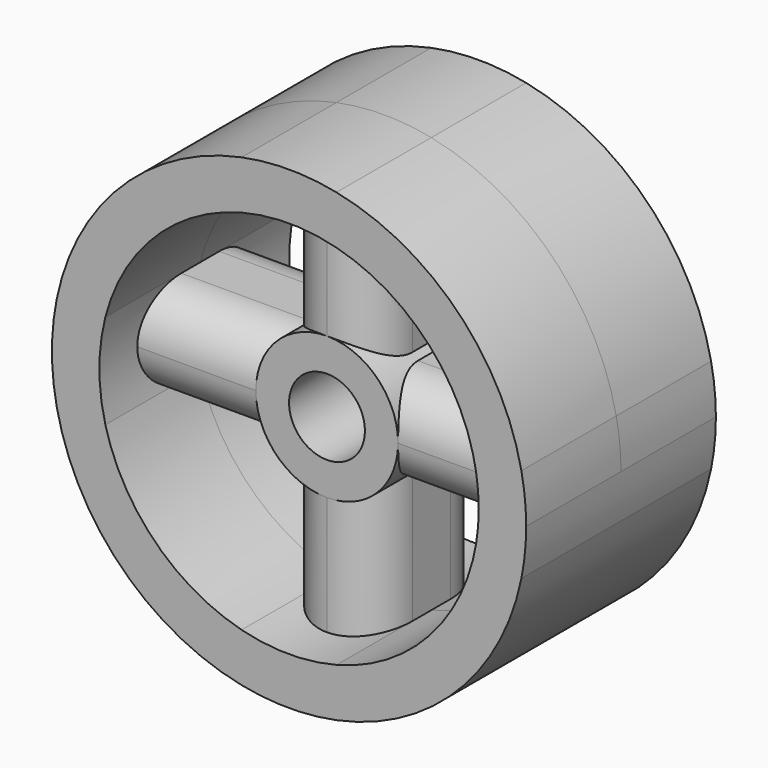
from build123d import *

# Parameters (mm, degrees)
F1_DEPTH = 12.5
F0_R     = 4
F2_DEPTH = 7.5
F3_R     = 4.99999
F4_R     = 4.99999


# Not quite as in the source:
# - a fillet or chamfer is up to 0.001 mm smaller than in the source, because OpenCascade refuses the exact size


with BuildPart() as f1:
    # F0 (on Front) → F1 (new body, symmetric)
    with BuildSketch(Plane.XZ):
        with BuildLine():
            ThreePointArc((24.4948974278, -5), (24.8734038251, -2.5127240501), (25, 0))
            ThreePointArc((25, 0), (24.8734038309, 2.5127239934), (24.4948974506, 4.9999998882))
            ThreePointArc((24.4948974506, 4.9999998882), (17.67766957, 17.6776694893), (5, 24.4948974278))
            ThreePointArc((5, 24.4948974278), (0, 25), (-5, 24.4948974278))
            ThreePointArc((-5, 24.4948974278), (-17.6776695297, 17.6776695297), (-24.4948974278, 5))
            ThreePointArc((-24.4948974278, 5), (-25, 5.7e-08), (-24.4948974506, -4.9999998882))
            ThreePointArc((-24.4948974506, -4.9999998882), (-17.67766957, -17.6776694893), (-5, -24.4948974278))
            ThreePointArc((-5, -24.4948974278), (-5.7e-08, -25), (4.9999998882, -24.4948974506))
            ThreePointArc((4.9999998882, -24.4948974506), (17.6776694893, -17.67766957), (24.4948974278, -5))
        make_face()
        with BuildLine():
            ThreePointArc((-5, -19.364916731), (-14.1421356645, -14.1421355829), (-19.3649167599, -4.9999998882))
            ThreePointArc((-19.3649167599, -4.9999998882), (-20, 5.77e-08), (-19.364916731, 5))
            ThreePointArc((-19.364916731, 5), (-14.1421356237, 14.1421356237), (-5, 19.364916731))
            ThreePointArc((-5, 19.364916731), (0, 20), (5, 19.364916731))
            ThreePointArc((5, 19.364916731), (14.1421356645, 14.1421355829), (19.3649167599, 4.9999998882))
            ThreePointArc((19.3649167599, 4.9999998882), (19.8405939326, 2.5200857924), (20, 0))
            ThreePointArc((20, 0), (19.8405939253, -2.5200858497), (19.364916731, -5))
            ThreePointArc((19.364916731, -5), (14.1421355829, -14.1421356645), (4.9999998882, -19.3649167599))
            ThreePointArc((4.9999998882, -19.3649167599), (-5.77e-08, -20), (-5, -19.364916731))
        make_face(mode=Mode.SUBTRACT)
    extrude(amount=F1_DEPTH, both=True)

    # F0 (on Front) → F2 (join, symmetric)
    with BuildSketch(Plane.XZ):
        with BuildLine():
            Line((-19.3649167599, -4.9999998882), (-5.5901700437, -4.9999998882))
            ThreePointArc((-5.5901700437, -4.9999998882), (-5.3033009119, -5.3033008059), (-5, -5.5901699437))
            Line((-5, -5.5901699437), (-5, -19.364916731))
            ThreePointArc((-5, -19.364916731), (-5.77e-08, -20), (4.9999998882, -19.3649167599))
            Line((4.9999998882, -19.3649167599), (4.9999998882, -5.5901700437))
            ThreePointArc((4.9999998882, -5.5901700437), (5.3033008059, -5.3033009119), (5.5901699437, -5))
            Line((5.5901699437, -5), (19.364916731, -5))
            ThreePointArc((19.364916731, -5), (19.8405939253, -2.5200858497), (20, 0))
            ThreePointArc((20, 0), (19.8405939326, 2.5200857924), (19.3649167599, 4.9999998882))
            Line((19.3649167599, 4.9999998882), (5.5901700437, 4.9999998882))
            ThreePointArc((5.5901700437, 4.9999998882), (5.3033009119, 5.3033008059), (5, 5.5901699437))
            Line((5, 5.5901699437), (5, 19.364916731))
            ThreePointArc((5, 19.364916731), (0, 20), (-5, 19.364916731))
            Line((-5, 19.364916731), (-5, 5.5901699437))
            ThreePointArc((-5, 5.5901699437), (-5.3033008589, 5.3033008589), (-5.5901699437, 5))
            Line((-5.5901699437, 5), (-19.364916731, 5))
            ThreePointArc((-19.364916731, 5), (-20, 5.77e-08), (-19.3649167599, -4.9999998882))
        make_face()
        Circle(F0_R, mode=Mode.SUBTRACT)
    extrude(amount=F2_DEPTH, both=True)

    # F3 (radius 5 in the source; OpenCascade refuses exactly that, so slightly less here)
    f3_edges = [f1.edges().sort_by_distance(p)[0] for p in [
        (12.477543, 7.5, 5),
    ]]
    fillet(f3_edges, radius=F3_R)

    # F4 (radius 5 in the source; OpenCascade refuses exactly that, so slightly less here)
    f4_edges = [f1.edges().sort_by_distance(p)[0] for p in [
        (12.477543, 7.5, -5),
        (-12.477543, 7.5, 5),
        (-12.477543, 7.5, -5),
        (-5, 7.5, -12.477543),
        (5, 7.5, -12.477543),
        (-5, 7.5, 12.477543),
        (5, 7.5, 12.477543),
        (12.477543, -7.5, 5),
        (12.477543, -7.5, -5),
        (5, -7.5, -12.477543),
        (-5, -7.5, -12.477543),
        (-12.477543, -7.5, -5),
        (-12.477543, -7.5, 5),
        (-5, -7.5, 12.477543),
        (5, -7.5, 12.477543),
    ]]
    fillet(f4_edges, radius=F4_R)


solid = f1.part
